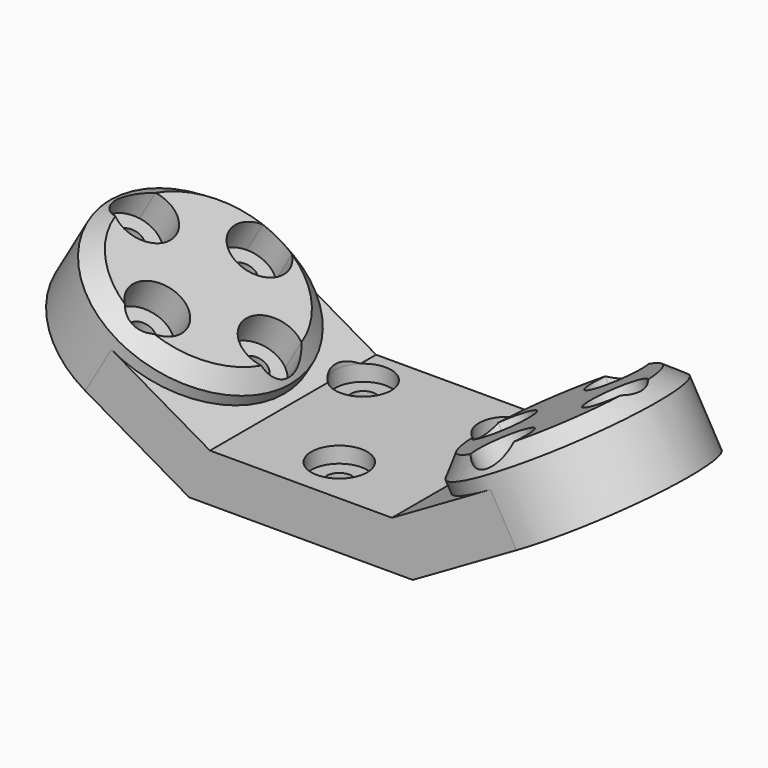
from build123d import *

# Parameters (mm, degrees)
F0_W      = 28
F0_H      = 26
F0_R      = 1.55
F1_DEPTH  = 6
F5_DEPTH  = 6.5
F6_DEPTH  = 10
F9_R      = 1.6
F10_DEPTH = 4
F11_DEPTH = 25
F12_START = -6
F9_R_2    = 3.5
F12_DEPTH = 19
F13_R     = 1.6
F14_DEPTH = 4
F15_DEPTH = 25
F16_START = -6
F13_R_2   = 3.5
F16_DEPTH = 19
F17_R     = 3.5
F18_DEPTH = 2
F19_DEPTH = 25


# Not quite as in the source:
# - a fillet or chamfer that OpenCascade refuses, or shapes differently, is made with other operations: its cross-section is extruded or revolved along the edge and cut away or added


with BuildPart() as f1:
    # F0 (on Top) → F1 (new body)
    with BuildSketch(Plane.XY):
        Rectangle(F0_W, F0_H)
        with Locations((0, -7)):
            Circle(F0_R, mode=Mode.SUBTRACT)
        with Locations((-9, 8)):
            Circle(F0_R, mode=Mode.SUBTRACT)
        with Locations((9, 8)):
            Circle(F0_R, mode=Mode.SUBTRACT)
    extrude(amount=F1_DEPTH)

    # F4 (on face) → F5 (join)
    with BuildSketch(Plane(origin=(3.5, 0, -6.0621778265), x_dir=(0.8660254038, 0, 0.5), z_dir=(-0.5, 0, 0.8660254038))):
        with BuildLine():
            Line((12.124355653, -13), (27.124355653, -13))
            ThreePointArc((27.124355653, -13), (14.124355653, 0), (27.124355653, 13))
            Line((27.124355653, 13), (12.124355653, 13))
            Line((12.124355653, 13), (12.124355653, -13))
        make_face()
        with BuildLine():
            ThreePointArc((27.124355653, 13), (14.124355653, 0), (27.124355653, -13))
            ThreePointArc((27.124355653, -13), (36.3167438084, -9.1923881554), (40.124355653, 0))
            ThreePointArc((40.124355653, 0), (36.3167438084, 9.1923881554), (27.124355653, 13))
        make_face()
    extrude(amount=F5_DEPTH)

    # F4 (on face) → F6 (join)
    with BuildSketch(Plane(origin=(3.5, 0, -6.0621778265), x_dir=(0.8660254038, 0, 0.5), z_dir=(-0.5, 0, 0.8660254038))):
        with BuildLine():
            ThreePointArc((27.124355653, 13), (14.124355653, 0), (27.124355653, -13))
            ThreePointArc((27.124355653, -13), (36.3167438084, -9.1923881554), (40.124355653, 0))
            ThreePointArc((40.124355653, 0), (36.3167438084, 9.1923881554), (27.124355653, 13))
        make_face()
    extrude(amount=F6_DEPTH)

    # F7: chamfer of 2 on 1 edges, made by hand

    # F7_s1 → F7_t2 (revolve, cut)
    with BuildSketch(Plane.XZ):
        with BuildLine():
            Line((34.3259853721, 20.9074977067), (31.4393864323, 21.6809595615))
            Line((31.4393864323, 21.6809595615), (31.4193864323, 21.7156005776))
            ThreePointArc((31.4193864323, 21.7156005776), (32.3381910048, 22.1807529184), (33.228711306, 22.694895054))
            Line((33.228711306, 22.694895054), (33.2833523221, 22.6802540378))
            ThreePointArc((33.2833523221, 22.6802540378), (33.7974944577, 21.7897337366), (34.3606263882, 20.9274977067))
            Line((34.3606263882, 20.9274977067), (34.3259853721, 20.9074977067))
        make_face()
    revolve(axis=Axis((21.9903810568, 0, 16.1602540378), (0.5, 0, -0.8660254038)), mode=Mode.SUBTRACT)

    # F8: F1 across plane


with BuildPart() as f1_1:
    add(f1.part)
    add(f1.part.mirror(Plane.YZ))

    # F9 (on face) → F10 (cut)
    with BuildSketch(Plane(origin=(-1.5, 0, 2.5980762114), x_dir=(0.8660254038, 0, 0.5), z_dir=(-0.5, 0, 0.8660254038))):
        with BuildLine():
            ThreePointArc((23.9821806278, -10.5416666667), (27.124355653, -11.0000000001), (30.2665306781, -10.5416666667))
            ThreePointArc((30.2665306781, -10.5416666667), (30.5337260192, -9.7913240209), (30.624355653, -9))
            ThreePointArc((30.624355653, -9), (26.3330316321, -5.5906296338), (23.9821806278, -10.5416666667))
        make_face()
        with Locations((27.124355653, -9)):
            Circle(F9_R, mode=Mode.SUBTRACT)
        with BuildLine():
            ThreePointArc((23.9821806278, -10.5416666667), (27.124355653, -12.5), (30.2665306781, -10.5416666667))
            ThreePointArc((30.2665306781, -10.5416666667), (27.124355653, -11.0000000001), (23.9821806278, -10.5416666667))
        make_face()
        with BuildLine():
            ThreePointArc((22.624355653, 0), (20.2336206122, 3.3195679312), (16.3274806529, 2.1041602206))
            ThreePointArc((16.3274806529, 2.1041602206), (16.1243556529, 0), (16.3274806529, -2.1041602206))
            ThreePointArc((16.3274806529, -2.1041602206), (20.2336206122, -3.3195679312), (22.624355653, 0))
        make_face()
        with Locations((19.124355653, 0)):
            Circle(F9_R, mode=Mode.SUBTRACT)
        with BuildLine():
            ThreePointArc((16.3274806529, -2.1041602206), (16.1243556529, 0), (16.3274806529, 2.1041602206))
            ThreePointArc((16.3274806529, 2.1041602206), (15.624355653, 0), (16.3274806529, -2.1041602206))
        make_face()
        with BuildLine():
            ThreePointArc((30.624355653, 9), (30.5337260192, 9.7913240209), (30.2665306781, 10.5416666667))
            ThreePointArc((30.2665306781, 10.5416666667), (27.124355653, 11.0000000001), (23.9821806278, 10.5416666667))
            ThreePointArc((23.9821806278, 10.5416666667), (26.3330316321, 5.5906296338), (30.624355653, 9))
        make_face()
        with Locations((27.124355653, 9)):
            Circle(F9_R, mode=Mode.SUBTRACT)
        with BuildLine():
            ThreePointArc((23.9821806278, 10.5416666667), (27.124355653, 11.0000000001), (30.2665306781, 10.5416666667))
            ThreePointArc((30.2665306781, 10.5416666667), (27.124355653, 12.5), (23.9821806278, 10.5416666667))
        make_face()
        with BuildLine():
            ThreePointArc((38.124355653, 0), (38.0734566435, 1.0569709078), (37.9212306531, 2.1041602206))
            ThreePointArc((37.9212306531, 2.1041602206), (31.624355653, 0), (37.9212306531, -2.1041602206))
            ThreePointArc((37.9212306531, -2.1041602206), (38.0734566435, -1.0569709078), (38.124355653, 0))
        make_face()
        with Locations((35.124355653, 0)):
            Circle(F9_R, mode=Mode.SUBTRACT)
        with BuildLine():
            ThreePointArc((37.9212306531, -2.1041602206), (38.4439235842, -1.1092649593), (38.624355653, 0))
            ThreePointArc((38.624355653, 0), (38.4439235842, 1.1092649593), (37.9212306531, 2.1041602206))
            ThreePointArc((37.9212306531, 2.1041602206), (38.0734566435, 1.0569709078), (38.124355653, 0))
            ThreePointArc((38.124355653, 0), (38.0734566435, -1.0569709078), (37.9212306531, -2.1041602206))
        make_face()
        with Locations((35.124355653, 0)):
            Circle(F9_R)
        with Locations((19.124355653, 0)):
            Circle(F9_R)
        with Locations((27.124355653, 9)):
            Circle(F9_R)
        with Locations((27.124355653, -9)):
            Circle(F9_R)
    extrude(amount=-F10_DEPTH, mode=Mode.SUBTRACT)

    # F9 (on face) → F11 (cut)
    with BuildSketch(Plane(origin=(-1.5, 0, 2.5980762114), x_dir=(0.8660254038, 0, 0.5), z_dir=(-0.5, 0, 0.8660254038))):
        with Locations((35.124355653, 0)):
            Circle(F9_R)
        with Locations((19.124355653, 0)):
            Circle(F9_R)
        with Locations((27.124355653, -9)):
            Circle(F9_R)
        with Locations((27.124355653, 9)):
            Circle(F9_R)
    extrude(amount=-F11_DEPTH, mode=Mode.SUBTRACT)

    # F9 (on face) → F12 (cut)
    with BuildSketch(Plane(origin=(-1.5, 0, 2.5980762114), x_dir=(0.8660254038, 0, 0.5), z_dir=(-0.5, 0, 0.8660254038)).offset(F12_START)):
        with Locations((27.124355653, 0)):
            Circle(F9_R_2)
    extrude(amount=-F12_DEPTH, mode=Mode.SUBTRACT)

    # F13 (on face) → F14 (cut)
    with BuildSketch(Plane(origin=(1.5, 0, 2.5980762114), x_dir=(0.8660254038, 0, -0.5), z_dir=(0.5, 0, 0.8660254038))):
        with BuildLine():
            ThreePointArc((-25.0201954324, -10.7968750001), (-23.9926978834, -9.56292022), (-23.624355653, -8))
            ThreePointArc((-23.624355653, -8), (-28.687275873, -4.8683422304), (-29.2285158736, -10.7968750001))
            ThreePointArc((-29.2285158736, -10.7968750001), (-27.124355653, -11.0000000001), (-25.0201954324, -10.7968750001))
        make_face()
        with Locations((-27.124355653, -8)):
            Circle(F13_R, mode=Mode.SUBTRACT)
        with BuildLine():
            ThreePointArc((-25.0201954324, 10.7968750001), (-27.124355653, 11.0000000001), (-29.2285158736, 10.7968750001))
            ThreePointArc((-29.2285158736, 10.7968750001), (-28.687275873, 4.8683422304), (-23.624355653, 8))
            ThreePointArc((-23.624355653, 8), (-23.9926978834, 9.56292022), (-25.0201954324, 10.7968750001))
        make_face()
        with Locations((-27.124355653, 8)):
            Circle(F13_R, mode=Mode.SUBTRACT)
        with BuildLine():
            ThreePointArc((-37.6660223197, 3.1421750251), (-38.124355653, 0), (-37.6660223197, -3.1421750251))
            ThreePointArc((-37.6660223197, -3.1421750251), (-34.2731173287, -2.9703394868), (-32.624355653, 0))
            ThreePointArc((-32.624355653, 0), (-34.2731173287, 2.9703394868), (-37.6660223197, 3.1421750251))
        make_face()
        with Locations((-36.124355653, 0)):
            Circle(F13_R, mode=Mode.SUBTRACT)
        with BuildLine():
            ThreePointArc((-16.5826889862, 3.1421750251), (-21.624355653, 0), (-16.5826889862, -3.1421750251))
            ThreePointArc((-16.5826889862, -3.1421750251), (-16.2395420731, -1.5877132403), (-16.1243556529, 0))
            ThreePointArc((-16.1243556529, 0), (-16.2395420731, 1.5877132403), (-16.5826889862, 3.1421750251))
        make_face()
        with Locations((-18.124355653, 0)):
            Circle(F13_R, mode=Mode.SUBTRACT)
        with Locations((-36.124355653, 0)):
            Circle(F13_R)
        with Locations((-18.124355653, 0)):
            Circle(F13_R)
        with Locations((-27.124355653, -8)):
            Circle(F13_R)
        with Locations((-27.124355653, 8)):
            Circle(F13_R)
        with BuildLine():
            ThreePointArc((-37.6660223197, 3.1421750251), (-39.624355653, 0), (-37.6660223197, -3.1421750251))
            ThreePointArc((-37.6660223197, -3.1421750251), (-38.124355653, 0), (-37.6660223197, 3.1421750251))
        make_face()
        with BuildLine():
            ThreePointArc((-16.1243556529, 0), (-16.2395420731, -1.5877132403), (-16.5826889862, -3.1421750251))
            ThreePointArc((-16.5826889862, -3.1421750251), (-15.1540161662, -1.8512383243), (-14.624355653, 0))
            ThreePointArc((-14.624355653, 0), (-15.1540161662, 1.8512383243), (-16.5826889862, 3.1421750251))
            ThreePointArc((-16.5826889862, 3.1421750251), (-16.2395420731, 1.5877132403), (-16.1243556529, 0))
        make_face()
        with BuildLine():
            ThreePointArc((-25.0201954324, -10.7968750001), (-27.124355653, -11.0000000001), (-29.2285158736, -10.7968750001))
            ThreePointArc((-29.2285158736, -10.7968750001), (-27.124355653, -11.5), (-25.0201954324, -10.7968750001))
        make_face()
        with BuildLine():
            ThreePointArc((-25.0201954324, 10.7968750001), (-27.124355653, 11.5), (-29.2285158736, 10.7968750001))
            ThreePointArc((-29.2285158736, 10.7968750001), (-27.124355653, 11.0000000001), (-25.0201954324, 10.7968750001))
        make_face()
    extrude(amount=-F14_DEPTH, mode=Mode.SUBTRACT)

    # F13 (on face) → F15 (cut)
    with BuildSketch(Plane(origin=(1.5, 0, 2.5980762114), x_dir=(0.8660254038, 0, -0.5), z_dir=(0.5, 0, 0.8660254038))):
        with Locations((-18.124355653, 0)):
            Circle(F13_R)
        with Locations((-27.124355653, -8)):
            Circle(F13_R)
        with Locations((-36.124355653, 0)):
            Circle(F13_R)
        with Locations((-27.124355653, 8)):
            Circle(F13_R)
    extrude(amount=-F15_DEPTH, mode=Mode.SUBTRACT)

    # F13 (on face) → F16 (cut)
    with BuildSketch(Plane(origin=(1.5, 0, 2.5980762114), x_dir=(0.8660254038, 0, -0.5), z_dir=(0.5, 0, 0.8660254038)).offset(F16_START)):
        with Locations((-27.124355653, 0)):
            Circle(F13_R_2)
    extrude(amount=-F16_DEPTH, mode=Mode.SUBTRACT)

    # F17 (on face) → F18 (cut)
    with BuildSketch(Plane.XY.offset(6)):
        with Locations((-9, 8)):
            Circle(F17_R)
        with Locations((9, 8)):
            Circle(F17_R)
        with Locations((0, -7)):
            Circle(F17_R)
    extrude(amount=-F18_DEPTH, mode=Mode.SUBTRACT)

    # F17 (on face) → F19 (cut)
    with BuildSketch(Plane.XY.offset(6)):
        with Locations((-9, 8)):
            Circle(F17_R)
        with Locations((9, 8)):
            Circle(F17_R)
        with Locations((0, -7)):
            Circle(F17_R)
    extrude(amount=F19_DEPTH, mode=Mode.SUBTRACT)


solid = f1_1.part
